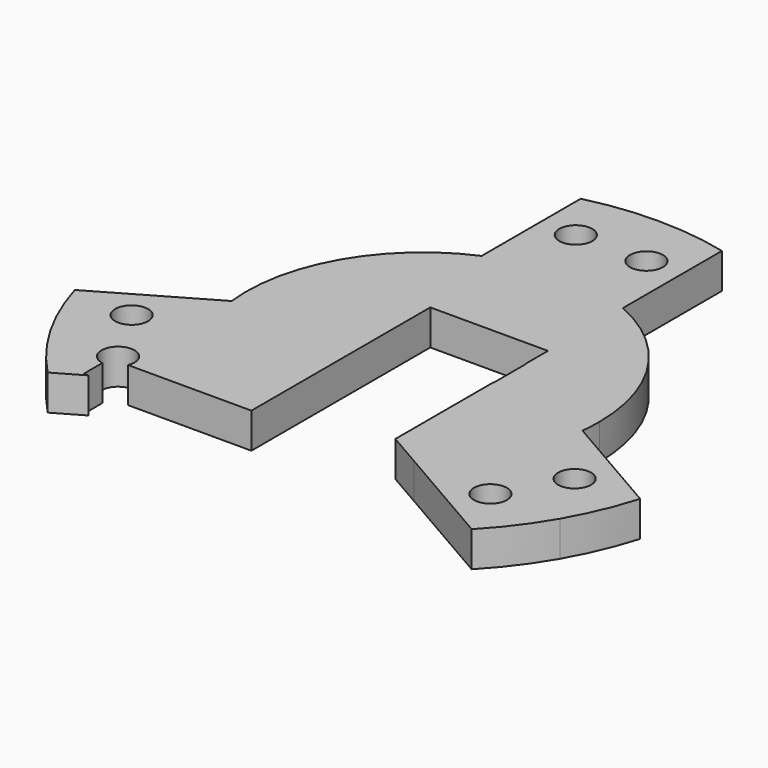
from build123d import *

# Parameters (mm, degrees)
F0_R     = 1.4019816861
F1_DEPTH = 3


with BuildPart() as f1:
    # F0 (on Top) → F1 (new body)
    with BuildSketch(Plane.XY):
        with BuildLine():
            Line((-18.017849557, -17.3308135222), (-24.017849557, -6.9385086768))
            ThreePointArc((-24.017849557, -6.9385086768), (-21.6506350946, -12.5), (-18.017849557, -17.3308135222))
        make_face()
        with BuildLine():
            Line((0, 25), (0, 24.269322199))
            Line((0, 24.269322199), (6, 24.269322199))
            ThreePointArc((6, 24.269322199), (3.0221635482, 24.8166582659), (0, 25))
        make_face()
        with BuildLine():
            Line((-6, 24.269322199), (0, 24.269322199))
            Line((0, 24.269322199), (0, 25))
            ThreePointArc((0, 25), (-3.0221635482, 24.8166582659), (-6, 24.269322199))
        make_face()
        with BuildLine():
            Line((0, 15), (0, 5.84))
            Line((0, 5.84), (5.96, 5.84))
            Line((5.96, 5.84), (5.96, 3.4871956259))
            Line((5.96, 3.4871956259), (6, 3.4641016151))
            Line((6, 3.4641016151), (6, 13.7477270849))
            ThreePointArc((6, 13.7477270849), (3.0646446553, 14.683594694), (0, 15))
        make_face()
        with BuildLine():
            Line((-4.04, 5.84), (0, 5.84))
            Line((0, 5.84), (0, 15))
            ThreePointArc((0, 15), (-3.0646446553, 14.683594694), (-6, 13.7477270849))
            Line((-6, 13.7477270849), (-6, 3.4641016151))
            Line((-6, 3.4641016151), (-14.9058808998, -1.6777111197))
            ThreePointArc((-14.9058808998, -1.6777111197), (-12.9903810568, -7.5), (-8.9058808998, -12.0700159651))
            Line((-8.9058808998, -12.0700159651), (-4.04, -9.2606983178))
            Line((-4.04, -9.2606983178), (-4.04, 0))
            Line((-4.04, 0), (-4.04, 4.5957081427))
            Line((-4.04, 4.5957081427), (-4.04, 5.84))
        make_face()
        with BuildLine():
            ThreePointArc((-6, 13.7477270849), (-3.0646446553, 14.683594694), (0, 15))
            Line((0, 15), (0, 24.269322199))
            Line((0, 24.269322199), (-6, 24.269322199))
            Line((-6, 24.269322199), (-6, 13.7477270849))
        make_face()
        with Locations((-3, 20)):
            Circle(F0_R, mode=Mode.SUBTRACT)
        with BuildLine():
            ThreePointArc((14.9058808998, -1.6777111197), (12.9903810568, -7.5), (8.9058808998, -12.0700159651))
            Line((8.9058808998, -12.0700159651), (18.0175705244, -17.3306524227))
            Line((18.0175705244, -17.3306524227), (24.0175705244, -6.9383475773))
            Line((24.0175705244, -6.9383475773), (14.9058808998, -1.6777111197))
        make_face()
        with Locations((15.8205080757, -12.5980762114)):
            Circle(F0_R, mode=Mode.SUBTRACT)
        with Locations((18.8205080757, -7.4019237886)):
            Circle(F0_R, mode=Mode.SUBTRACT)
        with BuildLine():
            Line((-10.7937886276, -13.16), (-8.9058808998, -12.0700159651))
            ThreePointArc((-8.9058808998, -12.0700159651), (-12.9903810568, -7.5), (-14.9058808998, -1.6777111197))
            Line((-14.9058808998, -1.6777111197), (-24.017849557, -6.9385086768))
            Line((-24.017849557, -6.9385086768), (-18.017849557, -17.3308135222))
            Line((-18.017849557, -17.3308135222), (-15.6435308888, -15.96))
            Line((-15.6435308888, -15.96), (-16.04, -15.96))
            Line((-16.04, -15.96), (-16.04, -13.9827696588))
            ThreePointArc((-16.04, -13.9827696588), (-16.7309554904, -11.5319438776), (-14.4185263896, -12.5980762114))
            ThreePointArc((-14.4185263896, -12.5980762114), (-14.4482255838, -12.8851187355), (-14.5360648874, -13.16))
            Line((-14.5360648874, -13.16), (-10.7937886276, -13.16))
        make_face()
        with Locations((-18.8205080757, -7.4019237886)):
            Circle(F0_R, mode=Mode.SUBTRACT)
        with BuildLine():
            Line((0, 24.269322199), (0, 15))
            ThreePointArc((0, 15), (3.0646446553, 14.683594694), (6, 13.7477270849))
            Line((6, 13.7477270849), (6, 24.269322199))
            Line((6, 24.269322199), (0, 24.269322199))
        make_face()
        with Locations((3, 20)):
            Circle(F0_R, mode=Mode.SUBTRACT)
        with BuildLine():
            Line((6, 0), (5.96, 0))
            Line((5.96, 0), (5.96, -10.3692108346))
            Line((5.96, -10.3692108346), (8.9058808998, -12.0700159651))
            ThreePointArc((8.9058808998, -12.0700159651), (12.9903810568, -7.5), (14.9058808998, -1.6777111197))
            Line((14.9058808998, -1.6777111197), (6, 3.4641016151))
            Line((6, 3.4641016151), (6, 0))
        make_face()
        with BuildLine():
            Line((6, 13.7477270849), (6, 3.4641016151))
            Line((6, 3.4641016151), (14.9058808998, -1.6777111197))
            ThreePointArc((14.9058808998, -1.6777111197), (14.9764517409, -0.8401745364), (15, 0))
            ThreePointArc((15, 0), (12.549900398, 8.2158383626), (6, 13.7477270849))
        make_face()
        with BuildLine():
            Line((-6, 3.4641016151), (-6, 13.7477270849))
            ThreePointArc((-6, 13.7477270849), (-12.9903810568, 7.5), (-14.9058808998, -1.6777111197))
            Line((-14.9058808998, -1.6777111197), (-6, 3.4641016151))
        make_face()
        with BuildLine():
            Line((24.0175705244, -6.9383475773), (18.0175705244, -17.3306524227))
            ThreePointArc((18.0175705244, -17.3306524227), (19.9806943206, -15.025575873), (21.6506348679, -12.5000003926))
            ThreePointArc((21.6506348679, -12.5000003926), (23.0028773953, -9.7910013475), (24.0175705244, -6.9383475773))
        make_face()
        with BuildLine():
            Line((-4.04, -11.16), (-4.04, -9.2606983178))
            Line((-4.04, -9.2606983178), (-8.9058808998, -12.0700159651))
            ThreePointArc((-8.9058808998, -12.0700159651), (-8.0704738939, -12.6438701009), (-7.1982220027, -13.16))
            Line((-7.1982220027, -13.16), (-4.04, -13.16))
            Line((-4.04, -13.16), (-4.04, -11.16))
        make_face()
        with BuildLine():
            ThreePointArc((-7.1982220027, -13.16), (-8.0704738939, -12.6438701009), (-8.9058808998, -12.0700159651))
            Line((-8.9058808998, -12.0700159651), (-10.7937886276, -13.16))
            Line((-10.7937886276, -13.16), (-7.1982220027, -13.16))
        make_face()
    extrude(amount=-F1_DEPTH)


solid = f1.part
